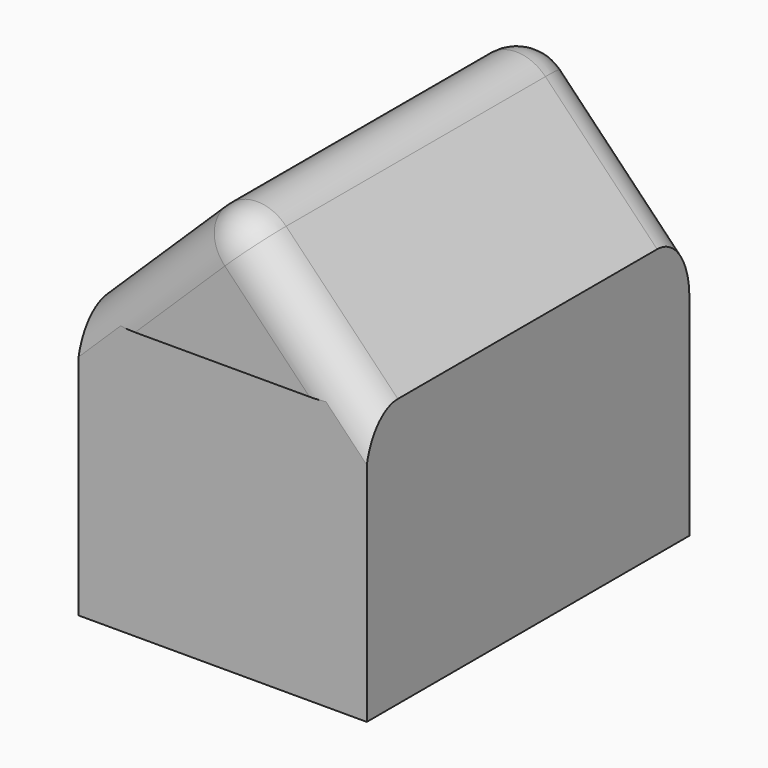
from build123d import *

# Parameters (mm, degrees)
F0_W         = 36.3061204553
F0_H         = 33.8365361094
F1_DEPTH     = 25.4
F5_DEPTH     = 50.99146
F7_T1_DEPTH  = 32.9564355705
F7_T3_DEPTH  = 33.7043488182
F7_T5_DEPTH  = 40.83146
F7_T10_DEPTH = 5.08
F7_T16_DEPTH = 5.08


# Not quite as in the source:
# - a fillet or chamfer that OpenCascade refuses, or shapes differently, is made with other operations: its cross-section is extruded or revolved along the edge and cut away or added
# - a feature of the source that left no trace in its solid (it failed there, or was rolled back) is left out


with BuildPart() as f1:
    # F0 (on Front) → F1 (new body, symmetric)
    with BuildSketch(Plane.XZ):
        with Locations((-18.1530602276, 16.9182680547)):
            Rectangle(F0_W, F0_H)
    extrude(amount=F1_DEPTH, both=True)

    # F3 (on face) → F5 (join)
    with BuildSketch(Plane(origin=(0, 25.4, 0), x_dir=(-1, 0, 0), z_dir=(0, 1, 0))):
        Polygon((36.3061204553, 33.8365361094), (17.6228713244, 52.0772151649), (0, 33.8365361094), align=None)
    extrude(amount=-F5_DEPTH)

    # F7: fillet of radius 5.08 on 5 edges, made by hand

    # F7_s2 → F7_t1 (cut)
    with BuildSketch(Plane(origin=(-30.9828597215, 0, 32.0690306362), x_dir=(0, 1, 0), z_dir=(0.6948226329, 0, -0.7191811377))):
        with BuildLine():
            ThreePointArc((-20.51146, 23.510391109), (-24.1035624484, 22.0224935574), (-25.59146, 18.430391109))
            Line((-25.59146, 18.430391109), (-25.59146, 23.510391109))
            Line((-25.59146, 23.510391109), (-20.51146, 23.510391109))
        make_face()
        with BuildLine():
            ThreePointArc((25.4, 18.430391109), (23.9121024484, 22.0224935574), (20.32, 23.510391109))
            Line((20.32, 23.510391109), (25.4, 23.510391109))
            Line((25.4, 23.510391109), (25.4, 18.430391109))
        make_face()
    extrude(amount=F7_T1_DEPTH, mode=Mode.SUBTRACT)

    # F7_s4 → F7_t3 (cut)
    with BuildSketch(Plane(origin=(-10.7619958041, 0, -10.507064916), x_dir=(0, 1, 0), z_dir=(0.7155307644, 0, 0.698581223))):
        with BuildLine():
            ThreePointArc((25.4, 44.4938565788), (23.9121024484, 48.0859590272), (20.32, 49.5738565788))
            Line((20.32, 49.5738565788), (25.4, 49.5738565788))
            Line((25.4, 49.5738565788), (25.4, 44.4938565788))
        make_face()
        with BuildLine():
            ThreePointArc((-20.51146, 49.5738565788), (-24.1035624484, 48.0859590272), (-25.59146, 44.4938565788))
            Line((-25.59146, 44.4938565788), (-25.59146, 49.5738565788))
            Line((-25.59146, 49.5738565788), (-20.51146, 49.5738565788))
        make_face()
    extrude(amount=F7_T3_DEPTH, mode=Mode.SUBTRACT)

    # F7_s6 → F7_t5 (cut)
    with BuildSketch(Plane.XZ.offset(-20.32)):
        with BuildLine():
            ThreePointArc((-14.074629897, 48.4045824879), (-17.6538784549, 49.9543417124), (-21.2768626893, 48.5097797958))
            Line((-21.2768626893, 48.5097797958), (-17.6228713244, 52.0772151649))
            Line((-17.6228713244, 52.0772151649), (-14.074629897, 48.4045824879))
        make_face()
    extrude(amount=F7_T5_DEPTH, mode=Mode.SUBTRACT)


with BuildPart() as f7_tool8:
    # F7_s9 → F7_t10 (new body)
    with BuildSketch(Plane.XZ.offset(20.51146)):
        Polygon((-17.7280700763, 44.8748835126), (-14.074629897, 48.4045824879), (-17.6228713244, 52.0772151649), (-21.2768626893, 48.5097797958), align=None)
    extrude(amount=F7_T10_DEPTH)

    # F7_s11 → F7_t12 (revolve, cut)
    with BuildSketch(Plane(origin=(-17.7280700763, -20.51146, 44.8748835126), x_dir=(-0.0146046499, 0, -0.9998933464), z_dir=(-0.9998933464, 0, 0.0146046499))):
        with BuildLine():
            ThreePointArc((0, -5.08), (5.08, 0), (0, 5.08))
            Line((0, 5.08), (0, -5.08))
        make_face()
    revolve(axis=Axis((-17.7280700763, -20.51146, 44.8748835126), (0, -1, 0)), mode=Mode.SUBTRACT)


with BuildPart() as f1_1:
    add(f1.part)

    # F7_t7: cut F7_tool8
    add(f7_tool8.part, mode=Mode.SUBTRACT)


with BuildPart() as f7_tool14:
    # F7_s15 → F7_t16 (new body)
    with BuildSketch(Plane.XZ.offset(-20.32)):
        Polygon((-17.7280700763, 44.8748835126), (-14.074629897, 48.4045824879), (-17.6228713244, 52.0772151649), (-21.2768626893, 48.5097797958), align=None)
    extrude(amount=-F7_T16_DEPTH)

    # F7_s17 → F7_t18 (revolve, cut)
    with BuildSketch(Plane(origin=(-17.7280700763, 20.32, 44.8748835126), x_dir=(-0.0146046499, 0, -0.9998933464), z_dir=(0.9998933464, 0, -0.0146046499))):
        with BuildLine():
            ThreePointArc((0, -5.08), (5.08, 0), (0, 5.08))
            Line((0, 5.08), (0, -5.08))
        make_face()
    revolve(axis=Axis((-17.7280700763, 20.32, 44.8748835126), (0, 1, 0)), mode=Mode.SUBTRACT)


with BuildPart() as f1_2:
    add(f1_1.part)

    # F7_t13: cut F7_tool14
    add(f7_tool14.part, mode=Mode.SUBTRACT)


solid = f1_2.part
